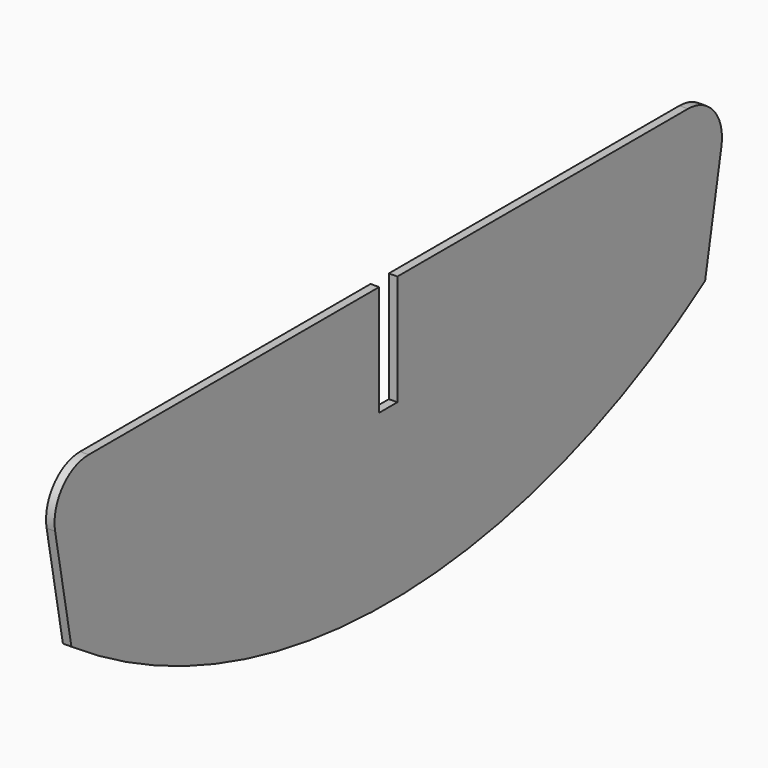
from build123d import *

# Parameters (mm, degrees)
F1_DEPTH = 1


# Not quite as in the source:
# - ends of sketch curves that miss each other by under 0.0002 mm in the source are joined


with BuildPart() as f1:
    # F0 (on Right) → F1 (new body)
    with BuildSketch(Plane.YZ):
        with BuildLine():
            Line((137.159267, 56.359386), (94.510204, 56.359386))
            ThreePointArc((94.510204, 56.359386), (90.6662324271, 54.5568666562), (89.5937941011, 50.4489390187))
            Line((89.5937941011, 50.4489390187), (91.984617, 37.538493))
            ThreePointArc((91.984617, 37.538493), (138.4992665872, 23.165856), (185.0139164157, 37.5384923916))
            Line((185.0139164157, 37.5384923916), (187.40474, 50.448939))
            ThreePointArc((187.40474, 50.448939), (186.3323015729, 54.5568666562), (182.48833, 56.359386))
            Line((182.48833, 56.359386), (139.839267, 56.359386))
            Line((139.839267, 56.359386), (139.839267, 43.359386))
            Line((139.839267, 43.359386), (137.159267, 43.359386))
            Line((137.159267, 43.359386), (137.159267, 56.359386))
        make_face()
    extrude(amount=F1_DEPTH)


solid = f1.part
